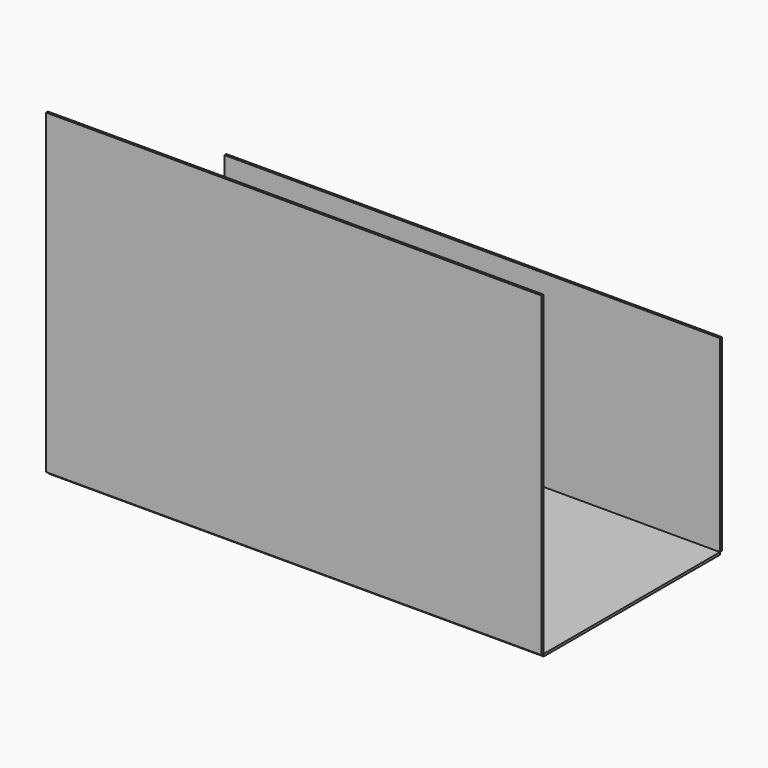
from build123d import *

# Parameters (mm, degrees)
F0_W     = 4025.9
F0_H     = 1790.7
F1_DEPTH = 19.05
F2_W     = 4025.9
F2_H     = 1530.35
F3_DEPTH = 19.05
F4_W     = 19.05
F4_H     = 2571.75
F5_DEPTH = 4025.9


# Not quite as in the source:
# - a feature names something its author has since deleted; it is built from what else it names


with BuildPart() as f1:
    # F0 (on Top) → F1 (new body)
    with BuildSketch(Plane.XY):
        with Locations((2012.95, -895.35)):
            Rectangle(F0_W, F0_H)
    extrude(amount=-F1_DEPTH)


with BuildPart() as f3:
    # F2 (on Front) → F3 (new body)
    with BuildSketch(Plane.XZ):
        with Locations((2012.95, 765.175)):
            Rectangle(F2_W, F2_H)
    extrude(amount=-F3_DEPTH)


with BuildPart() as f5:
    # F4 (on Right) → F5 (new body)
    with BuildSketch(Plane.YZ):
        with Locations((-1803.4116451339, 1285.875)):
            Rectangle(F4_W, F4_H)
    extrude(amount=F5_DEPTH)


solid = Compound([f1.part, f3.part, f5.part])
